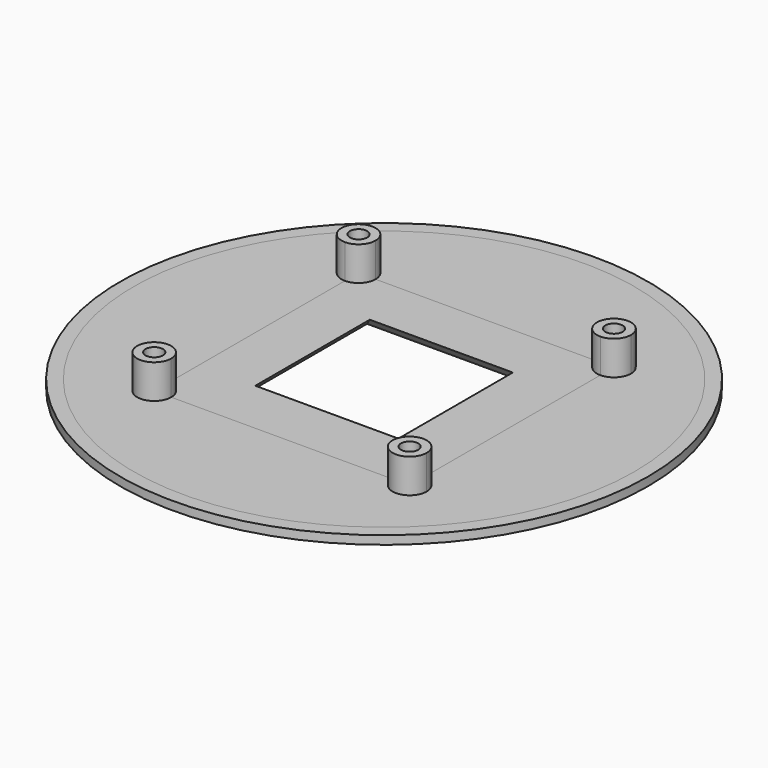
from build123d import *

# Parameters (mm, degrees)
F1_DEPTH         = 14
F0_W             = 40
F0_H             = 40
F2_DEPTH         = 4
F0_R             = 77.5
F0_R_2           = 73.549080942
F3_DEPTH         = 4
F4_DEPTH         = 4
F5_DEPTH         = 1.5
F6_D             = 5.1054
F6_CSINK_D       = 10.4394
F6_CSINK_ANGLE   = 82
F6_2_D           = 5.1054
F6_2_CSINK_D     = 10.4394
F6_2_CSINK_ANGLE = 82
F6_3_D           = 5.1054
F6_3_CSINK_D     = 10.4394
F6_3_CSINK_ANGLE = 82
F6_4_D           = 5.1054
F6_4_CSINK_D     = 10.4394
F6_4_CSINK_ANGLE = 82
F7_T1_DEPTH      = 40
F7_T3_DEPTH      = 40
F7_T9_DEPTH      = 52.8584149398
F7_T13_DEPTH     = 52.8584149398
F7_T20_DEPTH     = 52.8584149398
F7_T24_DEPTH     = 52.8584149398
F7_T31_DEPTH     = 52.8584149398
F7_T35_DEPTH     = 52.8584149398
F7_T42_DEPTH     = 52.8584149398
F7_T46_DEPTH     = 52.8584149398
F8_SIZE          = 1


# Not quite as in the source:
# - a fillet or chamfer that OpenCascade refuses, or shapes differently, is made with other operations: its cross-section is extruded or revolved along the edge and cut away or added


with BuildPart() as f1:
    # F0 (on Top) → F1 (new body)
    with BuildSketch(Plane.XY):
        with BuildLine():
            ThreePointArc((-32.5, -37.5), (-33.9644660941, -33.9644660941), (-37.5, -32.5))
            Line((-37.5, -32.5), (-37.5, -37.5))
            Line((-37.5, -37.5), (-32.5, -37.5))
        make_face()
        with BuildLine():
            Line((-37.5, -37.5), (-37.5, -32.5))
            ThreePointArc((-37.5, -32.5), (-41.0355339059, -41.0355339059), (-32.5, -37.5))
            Line((-32.5, -37.5), (-37.5, -37.5))
        make_face()
    extrude(amount=F1_DEPTH)

    # F6 (through all)
    with Locations(Plane(origin=(0, 0, 0), x_dir=(1, 0, 0), z_dir=(0, 0, -1))):
        with Locations((-37.5, -37.5), (37.5, -37.5), (37.5, 37.5), (-37.5, 37.5)):
            CounterSinkHole(F6_D / 2, F6_CSINK_D / 2, counter_sink_angle=F6_CSINK_ANGLE)


with BuildPart() as f1b:
    # F0 (on Top) → F1, piece 2 (new body)
    with BuildSketch(Plane.XY):
        with BuildLine():
            ThreePointArc((-37.5, 32.5), (-33.9644660941, 33.9644660941), (-32.5, 37.5))
            Line((-32.5, 37.5), (-37.5, 37.5))
            Line((-37.5, 37.5), (-37.5, 32.5))
        make_face()
        with BuildLine():
            Line((-37.5, 37.5), (-32.5, 37.5))
            ThreePointArc((-32.5, 37.5), (-41.0355339059, 41.0355339059), (-37.5, 32.5))
            Line((-37.5, 32.5), (-37.5, 37.5))
        make_face()
    extrude(amount=F1_DEPTH)

    # F6#2 (through all)
    with Locations(Plane(origin=(0, 0, 0), x_dir=(1, 0, 0), z_dir=(0, 0, -1))):
        with Locations((-37.5, -37.5), (37.5, -37.5), (37.5, 37.5), (-37.5, 37.5)):
            CounterSinkHole(F6_2_D / 2, F6_2_CSINK_D / 2, counter_sink_angle=F6_2_CSINK_ANGLE)


with BuildPart() as f1c:
    # F0 (on Top) → F1, piece 3 (new body)
    with BuildSketch(Plane.XY):
        with BuildLine():
            Line((37.5, -37.5), (37.5, -32.5))
            ThreePointArc((37.5, -32.5), (33.9644660941, -33.9644660941), (32.5, -37.5))
            Line((32.5, -37.5), (37.5, -37.5))
        make_face()
        with BuildLine():
            ThreePointArc((42.5, -37.5), (41.0355339059, -33.9644660941), (37.5, -32.5))
            Line((37.5, -32.5), (37.5, -37.5))
            Line((37.5, -37.5), (32.5, -37.5))
            ThreePointArc((32.5, -37.5), (37.5, -42.5), (42.5, -37.5))
        make_face()
    extrude(amount=F1_DEPTH)

    # F6#3 (through all)
    with Locations(Plane(origin=(0, 0, 0), x_dir=(1, 0, 0), z_dir=(0, 0, -1))):
        with Locations((-37.5, -37.5), (37.5, -37.5), (37.5, 37.5), (-37.5, 37.5)):
            CounterSinkHole(F6_3_D / 2, F6_3_CSINK_D / 2, counter_sink_angle=F6_3_CSINK_ANGLE)


with BuildPart() as f1d:
    # F0 (on Top) → F1, piece 4 (new body)
    with BuildSketch(Plane.XY):
        with BuildLine():
            Line((37.5, 37.5), (32.5, 37.5))
            ThreePointArc((32.5, 37.5), (33.9644660941, 33.9644660941), (37.5, 32.5))
            Line((37.5, 32.5), (37.5, 37.5))
        make_face()
        with BuildLine():
            ThreePointArc((42.5, 37.5), (37.5, 42.5), (32.5, 37.5))
            Line((32.5, 37.5), (37.5, 37.5))
            Line((37.5, 37.5), (37.5, 32.5))
            ThreePointArc((37.5, 32.5), (41.0355339059, 33.9644660941), (42.5, 37.5))
        make_face()
    extrude(amount=F1_DEPTH)

    # F6#4 (through all)
    with Locations(Plane(origin=(0, 0, 0), x_dir=(1, 0, 0), z_dir=(0, 0, -1))):
        with Locations((-37.5, -37.5), (37.5, -37.5), (37.5, 37.5), (-37.5, 37.5)):
            CounterSinkHole(F6_4_D / 2, F6_4_CSINK_D / 2, counter_sink_angle=F6_4_CSINK_ANGLE)


with BuildPart() as f2:
    # F0 (on Top) → F2 (new body)
    with BuildSketch(Plane.XY):
        with BuildLine():
            Line((32.5, 37.5), (-32.5, 37.5))
            ThreePointArc((-32.5, 37.5), (-33.9644660941, 33.9644660941), (-37.5, 32.5))
            Line((-37.5, 32.5), (-37.5, -32.5))
            ThreePointArc((-37.5, -32.5), (-33.9644660941, -33.9644660941), (-32.5, -37.5))
            Line((-32.5, -37.5), (32.5, -37.5))
            ThreePointArc((32.5, -37.5), (33.9644660941, -33.9644660941), (37.5, -32.5))
            Line((37.5, -32.5), (37.5, 32.5))
            ThreePointArc((37.5, 32.5), (33.9644660941, 33.9644660941), (32.5, 37.5))
        make_face()
        Rectangle(F0_W, F0_H, mode=Mode.SUBTRACT)
    extrude(amount=F2_DEPTH)

    # F7: chamfer of 5 on 4 edges, made by hand

    # F7_s2 → F7_t1 (cut)
    with BuildSketch(Plane.YZ.offset(-20)):
        Polygon((-20, 5), (-25, 0), (-20, 0), align=None)
        Polygon((20, 5), (25, 0), (20, 0), align=None)
    extrude(amount=F7_T1_DEPTH, mode=Mode.SUBTRACT)

    # F7_s4 → F7_t3 (cut)
    with BuildSketch(Plane.XZ.offset(-20)):
        Polygon((20, 5), (25, 0), (20, 0), align=None)
        Polygon((-20, 5), (-25, 0), (-20, 0), align=None)
    extrude(amount=F7_T3_DEPTH, mode=Mode.SUBTRACT)


with BuildPart() as f3:
    # F0 (on Top) → F3 (new body)
    with BuildSketch(Plane.XY):
        Circle(F0_R)
        Circle(F0_R_2, mode=Mode.SUBTRACT)
    extrude(amount=F3_DEPTH)

    # F0 (on Top) → F5 (cut)
    with BuildSketch(Plane.XY):
        Circle(F0_R)
        Circle(F0_R_2, mode=Mode.SUBTRACT)
    extrude(amount=F5_DEPTH, mode=Mode.SUBTRACT)


with BuildPart() as f4:
    # F0 (on Top) → F4 (new body)
    with BuildSketch(Plane.XY):
        Circle(F0_R_2)
        with BuildLine():
            ThreePointArc((-37.5, 32.5), (-41.0355339059, 41.0355339059), (-32.5, 37.5))
            Line((-32.5, 37.5), (32.5, 37.5))
            ThreePointArc((32.5, 37.5), (37.5, 42.5), (42.5, 37.5))
            ThreePointArc((42.5, 37.5), (41.0355339059, 33.9644660941), (37.5, 32.5))
            Line((37.5, 32.5), (37.5, -32.5))
            ThreePointArc((37.5, -32.5), (41.0355339059, -33.9644660941), (42.5, -37.5))
            ThreePointArc((42.5, -37.5), (37.5, -42.5), (32.5, -37.5))
            Line((32.5, -37.5), (-32.5, -37.5))
            ThreePointArc((-32.5, -37.5), (-41.0355339059, -41.0355339059), (-37.5, -32.5))
            Line((-37.5, -32.5), (-37.5, 32.5))
        make_face(mode=Mode.SUBTRACT)
    extrude(amount=F4_DEPTH)

    # F8
    f8_edges = [f4.edges().sort_by_distance(p)[0] for p in [
        (-73.549081, 0, 0),
    ]]
    chamfer(f8_edges, length=F8_SIZE)


with BuildPart() as f7_tool7:
    # F7_s8 → F7_t9 (new body)
    with BuildSketch(Plane.XZ.offset(-20)):
        Polygon((20, 5), (25, 0), (20, 0), align=None)
    extrude(amount=F7_T9_DEPTH)

    split(bisect_by=Plane.XZ.offset(20), keep=Keep.TOP)


with BuildPart() as f7_tool11:
    # F7_s12 → F7_t13 (new body)
    with BuildSketch(Plane.YZ.offset(32.8584149398)):
        Polygon((-20, 5), (-25, 0), (-20, 0), align=None)
    extrude(amount=-F7_T13_DEPTH)

    split(bisect_by=Plane.YZ.offset(20), keep=Keep.TOP)


with BuildPart() as f7_tool7_1:
    add(f7_tool7.part)

    # F7_t15: intersect F7_tool11
    add(f7_tool11.part, mode=Mode.INTERSECT)


with BuildPart() as f2_1:
    add(f2.part)

    # F7_t5: cut F7_tool7
    add(f7_tool7_1.part, mode=Mode.SUBTRACT)


with BuildPart() as f7_tool18:
    # F7_s19 → F7_t20 (new body)
    with BuildSketch(Plane.YZ.offset(20)):
        Polygon((-20, 5), (-25, 0), (-20, 0), align=None)
    extrude(amount=-F7_T20_DEPTH)

    split(bisect_by=Plane.YZ.offset(-20), keep=Keep.BOTTOM)


with BuildPart() as f7_tool22:
    # F7_s23 → F7_t24 (new body)
    with BuildSketch(Plane.XZ.offset(32.8584149398)):
        Polygon((-20, 5), (-25, 0), (-20, 0), align=None)
    extrude(amount=-F7_T24_DEPTH)

    split(bisect_by=Plane.XZ.offset(20), keep=Keep.TOP)


with BuildPart() as f7_tool18_1:
    add(f7_tool18.part)

    # F7_t26: intersect F7_tool22
    add(f7_tool22.part, mode=Mode.INTERSECT)


with BuildPart() as f2_2:
    add(f2_1.part)

    # F7_t16: cut F7_tool18
    add(f7_tool18_1.part, mode=Mode.SUBTRACT)


with BuildPart() as f7_tool29:
    # F7_s30 → F7_t31 (new body)
    with BuildSketch(Plane.XZ.offset(-32.8584149398)):
        Polygon((20, 5), (25, 0), (20, 0), align=None)
    extrude(amount=F7_T31_DEPTH)

    split(bisect_by=Plane.XZ.offset(-20), keep=Keep.BOTTOM)


with BuildPart() as f7_tool33:
    # F7_s34 → F7_t35 (new body)
    with BuildSketch(Plane.YZ.offset(-20)):
        Polygon((20, 5), (25, 0), (20, 0), align=None)
    extrude(amount=F7_T35_DEPTH)

    split(bisect_by=Plane.YZ.offset(20), keep=Keep.TOP)


with BuildPart() as f7_tool29_1:
    add(f7_tool29.part)

    # F7_t37: intersect F7_tool33
    add(f7_tool33.part, mode=Mode.INTERSECT)


with BuildPart() as f2_3:
    add(f2_2.part)

    # F7_t27: cut F7_tool29
    add(f7_tool29_1.part, mode=Mode.SUBTRACT)


with BuildPart() as f7_tool40:
    # F7_s41 → F7_t42 (new body)
    with BuildSketch(Plane.XZ.offset(20)):
        Polygon((-20, 5), (-25, 0), (-20, 0), align=None)
    extrude(amount=-F7_T42_DEPTH)

    split(bisect_by=Plane.XZ.offset(-20), keep=Keep.BOTTOM)


with BuildPart() as f7_tool44:
    # F7_s45 → F7_t46 (new body)
    with BuildSketch(Plane.YZ.offset(-32.8584149398)):
        Polygon((20, 5), (25, 0), (20, 0), align=None)
    extrude(amount=F7_T46_DEPTH)

    split(bisect_by=Plane.YZ.offset(-20), keep=Keep.BOTTOM)


with BuildPart() as f7_tool40_1:
    add(f7_tool40.part)

    # F7_t48: intersect F7_tool44
    add(f7_tool44.part, mode=Mode.INTERSECT)


with BuildPart() as f2_4:
    add(f2_3.part)

    # F7_t38: cut F7_tool40
    add(f7_tool40_1.part, mode=Mode.SUBTRACT)


solid = Compound([f1.part, f1b.part, f1c.part, f1d.part, f3.part, f4.part, f2_4.part])
